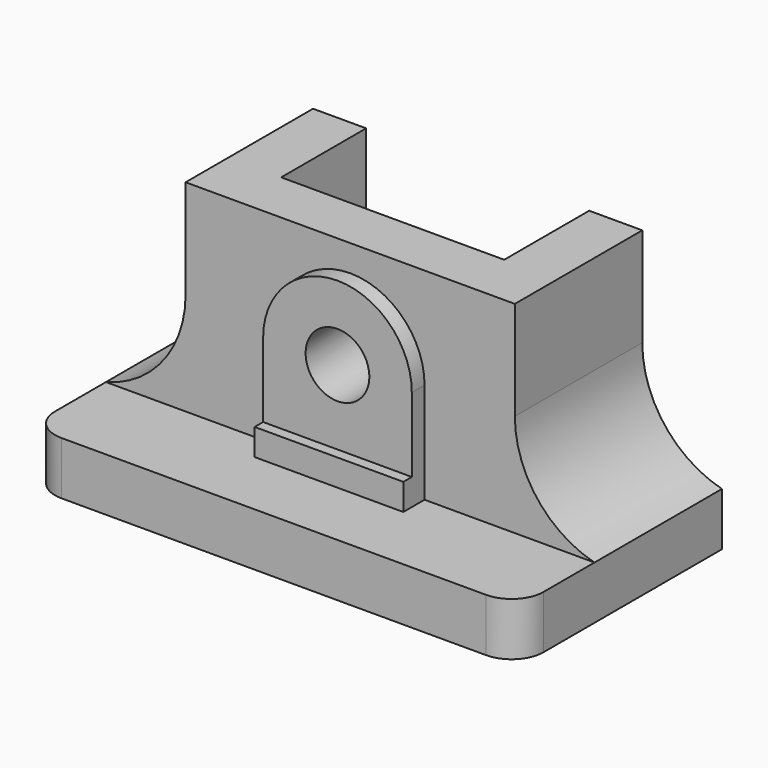
from build123d import *

# Parameters (mm, degrees)
F1_DEPTH    = 48
F2_DEPTH    = 10
F3_T1_DEPTH = 30
F4_T1_DEPTH = 30
F6_DEPTH    = 3
F5_W        = 28
F5_H        = 5
F7_DEPTH    = 5
F8_R        = 6
F9_R        = 6
F11_D       = 12


# Not quite as in the source:
# - a fillet or chamfer that OpenCascade refuses, or shapes differently, is made with other operations: its cross-section is extruded or revolved along the edge and cut away or added


with BuildPart() as f1:
    # F0 (on Top) → F1 (new body)
    with BuildSketch(Plane.XY):
        Polygon((-21, 20), (-31, 20), (-31, -10), (31, -10), (31, 20), (21, 20), (21, 0), (-21, 0), align=None)
    extrude(amount=F1_DEPTH)

    # F0 (on Top) → F2 (join)
    with BuildSketch(Plane.XY):
        Polygon((-31, 20), (-46, 20), (-46, -28), (46, -28), (46, 20), (31, 20), (31, -10), (-31, -10), align=None)
        Polygon((-21, 20), (-31, 20), (-31, -10), (31, -10), (31, 20), (21, 20), (21, 0), (-21, 0), align=None)
    extrude(amount=F2_DEPTH)

    # F3: fillet of radius 20 on 1 edges, made by hand

    # F3_s2 → F3_t1 (join)
    with BuildSketch(Plane.XZ.offset(-20)):
        with BuildLine():
            ThreePointArc((31, 29.364916731), (35.1886116992, 17.1174680171), (46, 10))
            Line((46, 10), (31, 10))
            Line((31, 10), (31, 29.364916731))
        make_face()
    extrude(amount=F3_T1_DEPTH)

    # F4: fillet of radius 20 on 1 edges, made by hand

    # F4_s2 → F4_t1 (join)
    with BuildSketch(Plane.XZ.offset(-20)):
        with BuildLine():
            ThreePointArc((-46, 10), (-35.1886116992, 17.1174680171), (-31, 29.364916731))
            Line((-31, 29.364916731), (-31, 10))
            Line((-31, 10), (-46, 10))
        make_face()
    extrude(amount=F4_T1_DEPTH)

    # F5 (on face) → F6 (join)
    with BuildSketch(Plane.XZ.offset(10)):
        with BuildLine():
            Line((-14, 29), (-14, 15))
            Line((-14, 15), (14, 15))
            Line((14, 15), (14, 29))
            ThreePointArc((14, 29), (0, 43), (-14, 29))
        make_face()
    extrude(amount=F6_DEPTH)

    # F5 (on face) → F7 (join)
    with BuildSketch(Plane.XZ.offset(10)):
        with Locations((0, 12.5)):
            Rectangle(F5_W, F5_H)
    extrude(amount=F7_DEPTH)

    # F8
    f8_edges = [f1.edges().sort_by_distance(p)[0] for p in [
        (46, -28, 5),
    ]]
    fillet(f8_edges, radius=F8_R)

    # F9
    f9_edges = [f1.edges().sort_by_distance(p)[0] for p in [
        (-46, -28, 5),
    ]]
    fillet(f9_edges, radius=F9_R)

    # F11 (through all)
    with Locations(Plane.XZ.offset(13)):
        with Locations((0, 29)):
            Hole(F11_D / 2)


solid = f1.part
